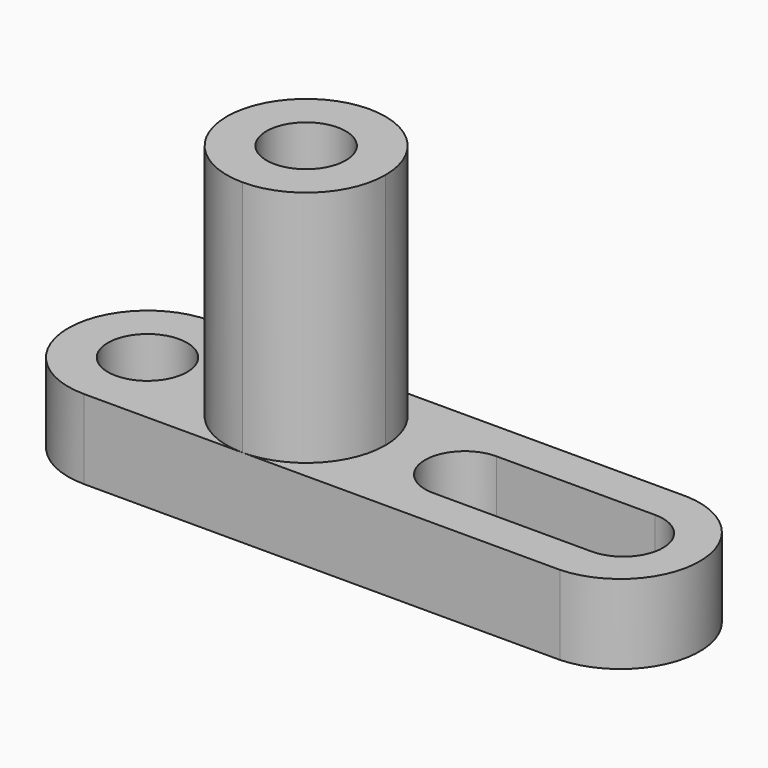
from build123d import *

# Parameters (mm, degrees)
F0_W      = 101.6
F0_H      = 12.7
F1_DEPTH  = 25.4
F2_R      = 6.35
F3_DEPTH  = 25.4
F5_DEPTH  = 25.4
F7_DEPTH  = 25.4
F9_DEPTH  = 38.1
F10_R     = 6.35
F11_DEPTH = 38.1
F13_DEPTH = 25.4


# Not quite as in the source:
# - ends of sketch curves that miss each other by under 0.0002 mm in the source are joined


with BuildPart() as f1:
    # F0 (on Front) → F1 (new body)
    with BuildSketch(Plane.XZ):
        with Locations((50.8, 6.35)):
            Rectangle(F0_W, F0_H)
    extrude(amount=F1_DEPTH)

    # F2 (on face) → F3 (cut)
    with BuildSketch(Plane.XY.offset(12.7)):
        with Locations((12.7, -12.7)):
            Circle(F2_R)
    extrude(amount=-F3_DEPTH, mode=Mode.SUBTRACT)

    # F4 (on face) → F5 (cut)
    with BuildSketch(Plane.XY.offset(12.7)):
        with BuildLine():
            ThreePointArc((-1.0081e-06, -12.7), (3.7197432273, -3.7197435225), (12.7, 0))
            Line((12.7, 0), (0, 0))
            Line((0, 0), (-1.0081e-06, -12.7))
        make_face()
        with BuildLine():
            ThreePointArc((12.6999979839, -25.4), (3.7197425145, -21.6802557647), (-1.0081e-06, -12.7))
            Line((-1.0081e-06, -12.7), (0, -25.4))
            Line((0, -25.4), (12.6999979839, -25.4))
        make_face()
    extrude(amount=-F5_DEPTH, mode=Mode.SUBTRACT)

    # F6 (on face) → F7 (cut)
    with BuildSketch(Plane.XY.offset(12.7)):
        with BuildLine():
            ThreePointArc((63.5, -6.35), (67.9901280605, -8.2098719395), (69.85, -12.7))
            ThreePointArc((69.85, -12.7), (67.9901280605, -17.1901280605), (63.5, -19.05))
            Line((63.5, -19.05), (88.9, -19.05))
            ThreePointArc((88.9, -19.05), (82.55, -12.7), (88.9, -6.35))
            Line((88.9, -6.35), (63.5, -6.35))
        make_face()
        with BuildLine():
            ThreePointArc((63.5, -19.05), (67.9901280605, -17.1901280605), (69.85, -12.7))
            ThreePointArc((69.85, -12.7), (67.9901280605, -8.2098719395), (63.5, -6.35))
            ThreePointArc((63.5, -6.35), (57.15, -12.7), (63.5, -19.05))
        make_face()
        with BuildLine():
            ThreePointArc((95.25, -12.7), (93.3901280605, -8.2098719395), (88.9, -6.35))
            ThreePointArc((88.9, -6.35), (82.55, -12.7), (88.9, -19.05))
            ThreePointArc((88.9, -19.05), (93.3901280605, -17.1901280605), (95.25, -12.7))
        make_face()
    extrude(amount=-F7_DEPTH, mode=Mode.SUBTRACT)

    # F8 (on face) → F9 (join)
    with BuildSketch(Plane.XY.offset(12.7)):
        with BuildLine():
            ThreePointArc((38.1, -25.4), (47.0802561211, -21.6802561211), (50.8, -12.7))
            ThreePointArc((50.8, -12.7), (47.0802561211, -3.7197438789), (38.1, 0))
            ThreePointArc((38.1, 0), (25.4, -12.7), (38.1, -25.4))
        make_face()
    extrude(amount=F9_DEPTH)

    # F10 (on face) → F11 (cut)
    with BuildSketch(Plane.XY.offset(50.8)):
        with Locations((38.1, -12.7)):
            Circle(F10_R)
    extrude(amount=-F11_DEPTH, mode=Mode.SUBTRACT)

    # F12 (on face) → F13 (cut)
    with BuildSketch(Plane.XY.offset(12.7)):
        with BuildLine():
            ThreePointArc((88.9, 0), (101.1192301161, -12.7), (88.9, -25.4))
            Line((88.9, -25.4), (101.6, -25.4))
            Line((101.6, -25.4), (101.6, 0))
            Line((101.6, 0), (88.9, 0))
        make_face()
    extrude(amount=-F13_DEPTH, mode=Mode.SUBTRACT)


solid = f1.part
